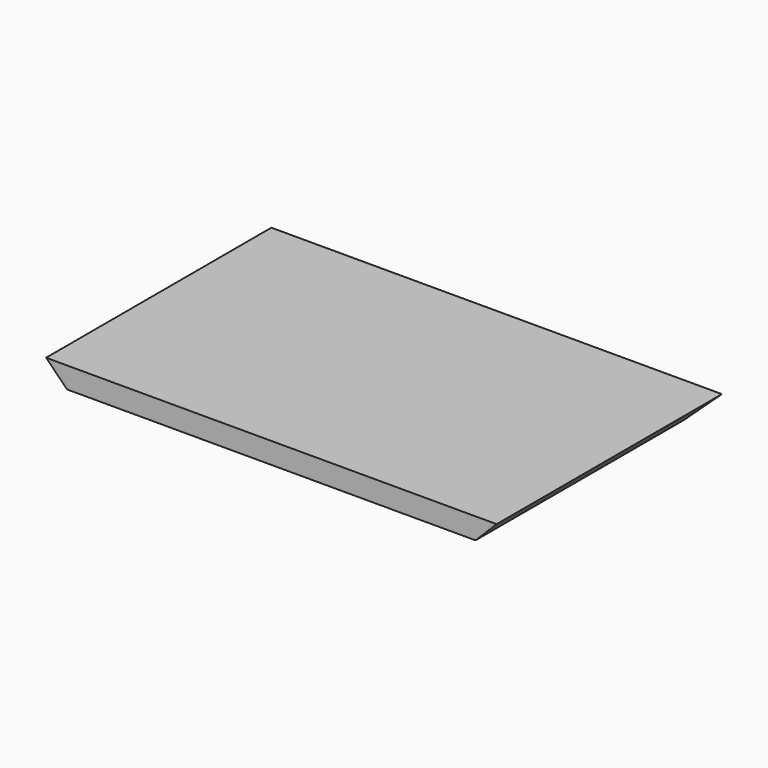
from build123d import *

# Parameters (mm, degrees)
F1_DEPTH = 254
F2_SIZE  = 19.04999
F3_W     = 63.5
F3_H     = 19.05
F4_DEPTH = 6.35


# Not quite as in the source:
# - a fillet or chamfer is up to 0.001 mm smaller than in the source, because OpenCascade refuses the exact size


with BuildPart() as f1:
    # F0 (on Front) → F1 (new body)
    with BuildSketch(Plane.XZ):
        Polygon((203.2, 9.525), (-203.2, 9.525), (-184.15, -9.525), (184.15, -9.525), align=None)
    extrude(amount=-F1_DEPTH)

    # F2 (size 19.05 in the source; OpenCascade refuses exactly that, so slightly less here)
    f2_edges = [f1.edges().sort_by_distance(p)[0] for p in [
        (0, 254, -9.525),
    ]]
    chamfer(f2_edges, length=F2_SIZE)

    # F3 (on face) → F4 (cut)
    with BuildSketch(Plane(origin=(0, 0, -9.525), x_dir=(1, 0, 0), z_dir=(0, 0, -1))):
        with Locations((-31.75, -206.375)):
            Rectangle(F3_W, F3_H)
        with Locations((-31.75, -28.575)):
            Rectangle(F3_W, F3_H)
        with Locations((152.4, -28.575)):
            Rectangle(F3_W, F3_H)
        with Locations((152.4, -206.375)):
            Rectangle(F3_W, F3_H)
    extrude(amount=-F4_DEPTH, mode=Mode.SUBTRACT)


solid = f1.part
